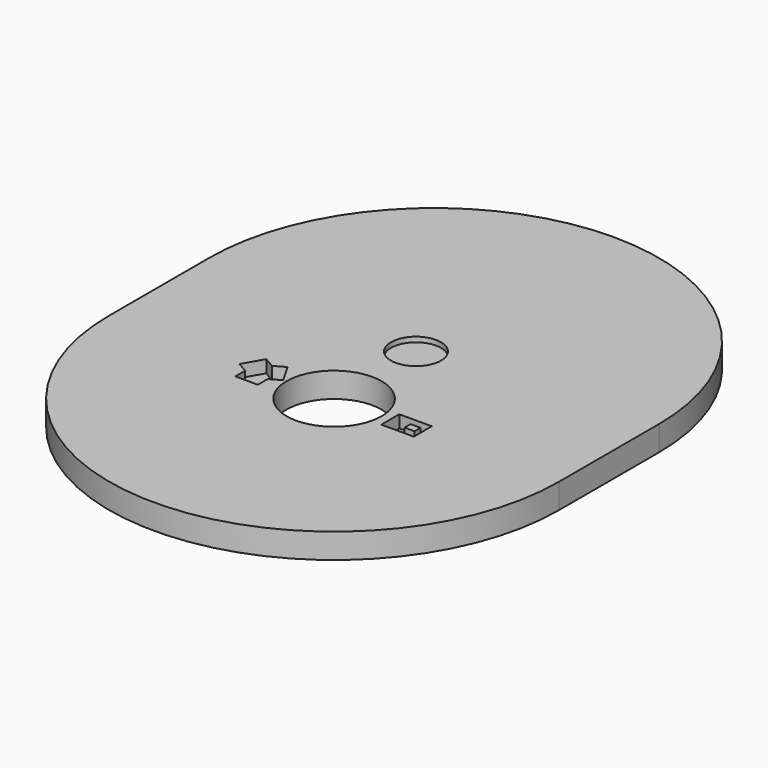
from build123d import *

# Parameters (mm, degrees)
F1_DEPTH  = 5
F3_DEPTH  = 2.5
F4_W      = 6.5
F4_H      = 4.5
F5_DEPTH  = 2.5
F6_W      = 2
F6_H      = 1.5
F7_DEPTH  = 1.5
F8_R      = 5
F9_DEPTH  = 1
F10_R     = 9.5
F11_DEPTH = 10
F14_DEPTH = 2.5
F12_R     = 5
F15_DEPTH = 1
F16_W     = 6.5
F16_H     = 4.5
F17_DEPTH = 2.5
F18_W     = 2
F18_H     = 1.5
F19_DEPTH = 1.5
F20_R     = 44.99999


# Not quite as in the source:
# - a fillet or chamfer is up to 0.001 mm smaller than in the source, because OpenCascade refuses the exact size


with BuildPart() as f1:
    # F0 (on Top) → F1 (new body)
    with BuildSketch(Plane.XY):
        with BuildLine():
            Line((-45, 70), (-45, 0))
            ThreePointArc((-45, 0), (0, -45), (45, 0))
            Line((45, 0), (45, 70))
            Line((45, 70), (-45, 70))
        make_face()
    extrude(amount=F1_DEPTH)

    # F2 (on face) → F3 (cut)
    with BuildSketch(Plane.XY.offset(5)):
        Polygon((-14.5, 2.6008529611), (-16.625, 3.8277222831), (-18.875, -0.0693920339), (-16.75, -1.2962613559), (-16.75, -3.75), (-12.25, -3.75), (-12.25, -1.2962613559), (-10.125, -0.0693920339), (-12.375, 3.8277222831), align=None)
    extrude(amount=-F3_DEPTH, mode=Mode.SUBTRACT)

    # F4 (on face) → F5 (cut)
    with BuildSketch(Plane.XY.offset(5)):
        with Locations((14.5, 0)):
            Rectangle(F4_W, F4_H)
    extrude(amount=-F5_DEPTH, mode=Mode.SUBTRACT)

    # F6 (on face) → F7 (join)
    with BuildSketch(Plane.XY.offset(2.5)):
        with Locations((14.5, 1.5)):
            Rectangle(F6_W, F6_H)
        with Locations((14.5, -1.5)):
            Rectangle(F6_W, F6_H)
    extrude(amount=F7_DEPTH)

    # F8 (on face) → F9 (cut)
    with BuildSketch(Plane.XY.offset(5)):
        with Locations((0, 20.4880452948)):
            Circle(F8_R)
    extrude(amount=-F9_DEPTH, mode=Mode.SUBTRACT)

    # F10 (on face) → F11 (cut)
    with BuildSketch(Plane(origin=(0, 0, 0), x_dir=(1, 0, 0), z_dir=(0, 0, -1))):
        Circle(F10_R)
    extrude(amount=-F11_DEPTH, mode=Mode.SUBTRACT)

    # F13 (on face) → F14 (cut)
    with BuildSketch(Plane(origin=(0, 0, 0), x_dir=(1, 0, 0), z_dir=(0, 0, -1))):
        Polygon((20, 32.6008529611), (17.875, 33.8277222831), (15.625, 29.9306079661), (17.75, 28.7037386441), (17.75, 26.25), (22.25, 26.25), (22.25, 28.7037386441), (24.375, 29.9306079661), (22.125, 33.8277222831), align=None)
    extrude(amount=-F14_DEPTH, mode=Mode.SUBTRACT)

    # F12 (on face) → F15 (cut)
    with BuildSketch(Plane(origin=(0, 0, 0), x_dir=(1, 0, 0), z_dir=(0, 0, -1))):
        with Locations((0, -60)):
            Circle(F12_R)
    extrude(amount=-F15_DEPTH, mode=Mode.SUBTRACT)

    # F16 (on face) → F17 (cut)
    with BuildSketch(Plane(origin=(0, 0, 0), x_dir=(1, 0, 0), z_dir=(0, 0, -1))):
        with Locations((-20, 30)):
            Rectangle(F16_W, F16_H)
    extrude(amount=-F17_DEPTH, mode=Mode.SUBTRACT)

    # F18 (on face) → F19 (join)
    with BuildSketch(Plane(origin=(0, 0, 2.5), x_dir=(1, 0, 0), z_dir=(0, 0, -1))):
        with Locations((-20, 31.5)):
            Rectangle(F18_W, F18_H)
        with Locations((-20, 28.5)):
            Rectangle(F18_W, F18_H)
    extrude(amount=F19_DEPTH)

    # F20 (radius 45 in the source; OpenCascade refuses exactly that, so slightly less here)
    f20_edges = [f1.edges().sort_by_distance(p)[0] for p in [
        (-45, 70, 2.5),
        (45, 70, 2.5),
    ]]
    fillet(f20_edges, radius=F20_R)


solid = f1.part
